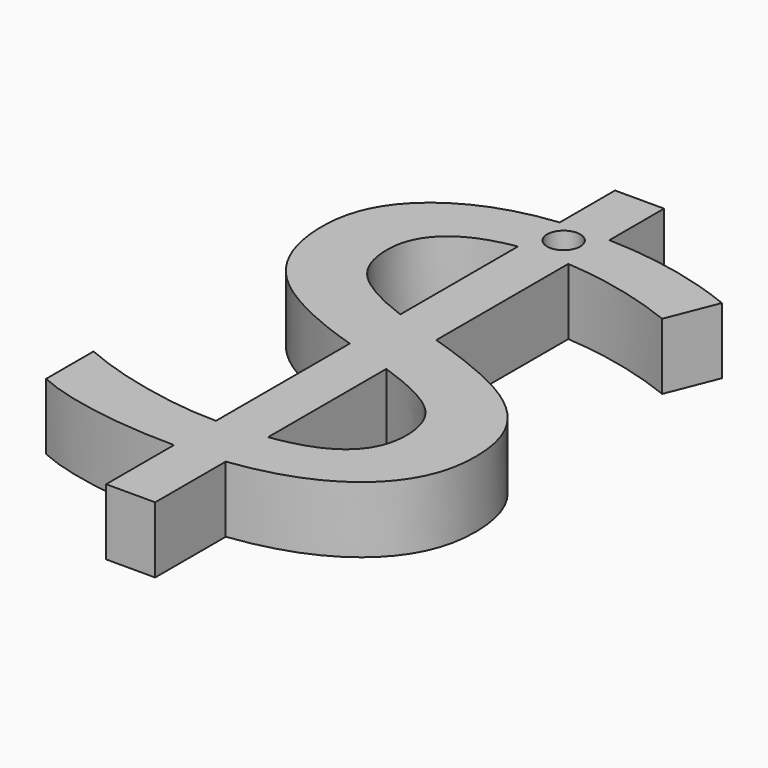
from build123d import *

# Parameters (mm, degrees)
F0_TEXT_SIZE = 59.7471681734
F1_DEPTH     = 5.08
F2_R         = 1.27
F3_DEPTH     = 14.478


# Not quite as in the source:
# - Text() gives the source's letters only with a copy of the font that has no kerning and outlines rounded to 1/6400 em; it was checked with that copy


with BuildPart() as f1:
    # F0 (on Top) → F1 (new body)
    with BuildSketch(Plane.XY):
        with Locations((0, 0)):
            Text('$', F0_TEXT_SIZE, font='Open Sans', text_align=(TextAlign.LEFT, TextAlign.BOTTOM))
    extrude(amount=F1_DEPTH)

    # F2 (on face) → F3 (cut)
    with BuildSketch(Plane.XY.offset(5.08)):
        with Locations((16.815058887, 38.354434073)):
            Circle(F2_R)
    extrude(amount=-F3_DEPTH, mode=Mode.SUBTRACT)


solid = f1.part
